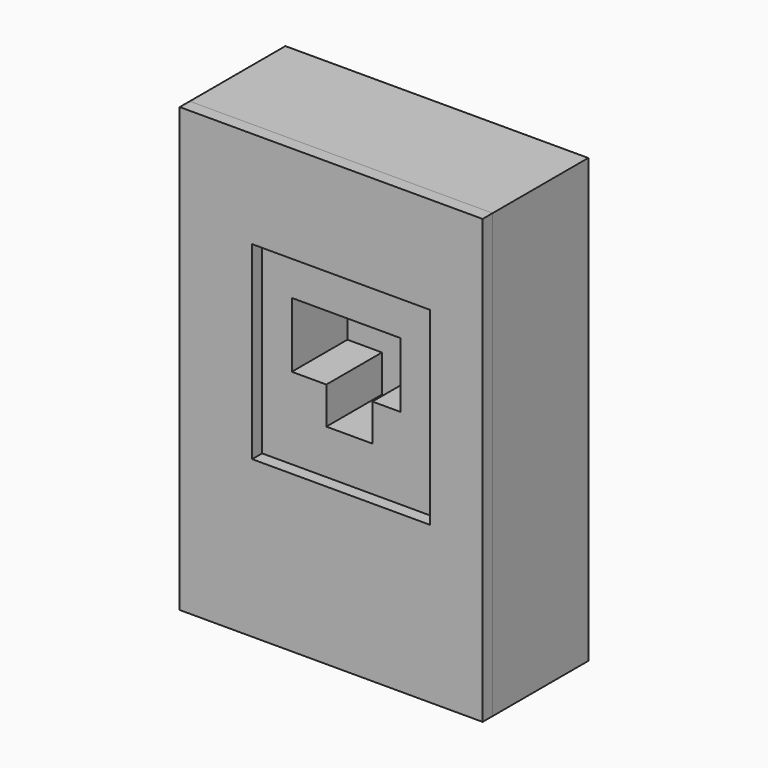
from build123d import *

# Parameters (mm, degrees)
F0_W     = 55.3452633321
F0_H     = 80.9123702347
F1_DEPTH = 21.844
F3_DEPTH = 12.7
F4_W     = 55.3452633321
F4_H     = 80.9123702347
F5_DEPTH = 2.286
F6_W     = 32.4852615595
F6_H     = 34.5907891169
F7_DEPTH = 25.4


with BuildPart() as f1:
    # F0 (on Front) → F1 (new body)
    with BuildSketch(Plane.XZ):
        with Locations((-0.7519740611, -3.0078943819)):
            Rectangle(F0_W, F0_H)
    extrude(amount=F1_DEPTH)

    # F2 (on face) → F3 (cut)
    with BuildSketch(Plane.XZ.offset(21.844)):
        Polygon((10.07644739, 11.8811847642), (-9.7756581381, 11.8811847642), (-9.7756581381, 0), (-3.4590791911, 0), (-3.4590791911, -6.7677632906), (4.9630273134, -6.7677632906), (4.9630273134, 0), (10.07644739, 0), align=None)
    extrude(amount=-F3_DEPTH, mode=Mode.SUBTRACT)


with BuildPart() as f5:
    # F4 (on face) → F5 (new body)
    with BuildSketch(Plane.XZ.offset(21.844)):
        with Locations((-0.7519740611, -3.0078943819)):
            Rectangle(F4_W, F4_H)
    extrude(amount=F5_DEPTH)

    # F6 (on face) → F7 (cut)
    with BuildSketch(Plane.XZ.offset(24.13)):
        with Locations((1.0527633131, 2.4063154124)):
            Rectangle(F6_W, F6_H)
    extrude(amount=-F7_DEPTH, mode=Mode.SUBTRACT)


solid = Compound([f1.part, f5.part])
